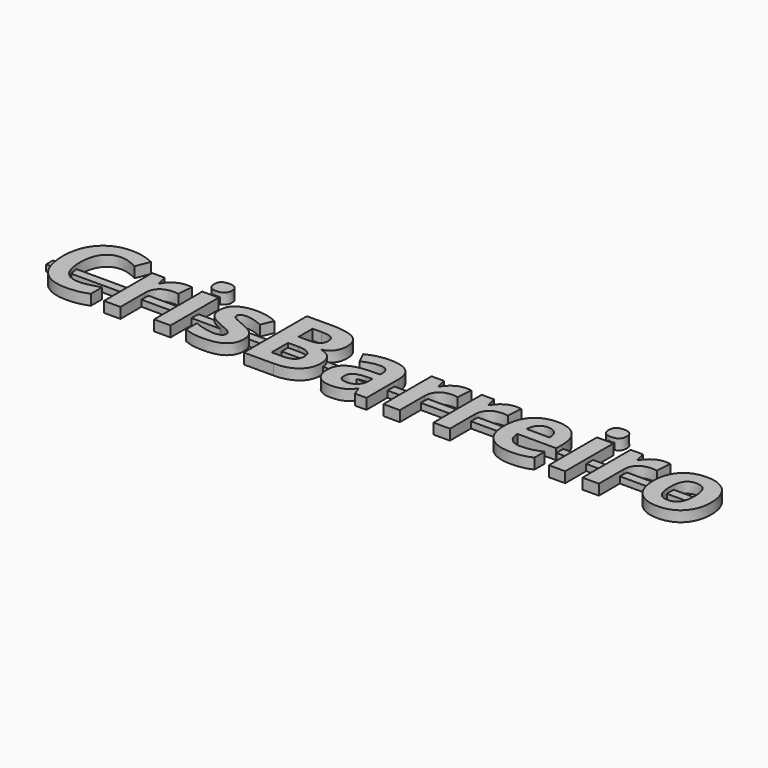
from build123d import *

# Parameters (mm, degrees)
F0_TEXT_SIZE = 10.4166666667
F1_DEPTH     = 1
F2_W         = 61.964508146
F2_H         = 0.8111610077
F3_DEPTH     = 0.6
F4_W         = 0.3
F4_H         = 2.6677125082
F5_DEPTH     = 0.6
F6_W         = 0.3
F6_H         = 2.3556580816
F6_W_2       = 0.2952529245
F7_DEPTH     = 0.6


# Not quite as in the source:
# - Text() gives the source's letters only with a copy of the font that has no kerning and outlines rounded to 1/6400 em; it was checked with that copy


with BuildPart() as f1:
    # F0 (on Top) → F1 (new body)
    with BuildSketch(Plane.XY):
        with Locations((0, -7.5)):
            Text('CrisBarreiro', F0_TEXT_SIZE, font='Open Sans', font_style=FontStyle.BOLD, text_align=(TextAlign.LEFT, TextAlign.BOTTOM))
    extrude(amount=F1_DEPTH)

    # F2 (on Top) → F3 (join)
    with BuildSketch(Plane.XY):
        with Locations((30.982254073, -4.6134449076)):
            Rectangle(F2_W, F2_H)
    extrude(amount=F3_DEPTH)

    # F4 (on face) → F5 (join)
    with BuildSketch(Plane(origin=(0, 0, 0), x_dir=(1, 0, 0), z_dir=(0, 0, -1))):
        with Locations((12.808984375, 1.6543669148)):
            Rectangle(F4_W, F4_H)
        with Locations((13.108984375, 1.6543669148)):
            Rectangle(F4_W, F4_H)
    extrude(amount=-F5_DEPTH)

    # F6 (on face) → F7 (join)
    with BuildSketch(Plane(origin=(0, 0, 0), x_dir=(1, 0, 0), z_dir=(0, 0, -1))):
        with Locations((50.0831951323, 1.4407557338)):
            Rectangle(F6_W, F6_H)
        with Locations((50.3808215946, 1.4407557338)):
            Rectangle(F6_W_2, F6_H)
    extrude(amount=-F7_DEPTH)


solid = f1.part
